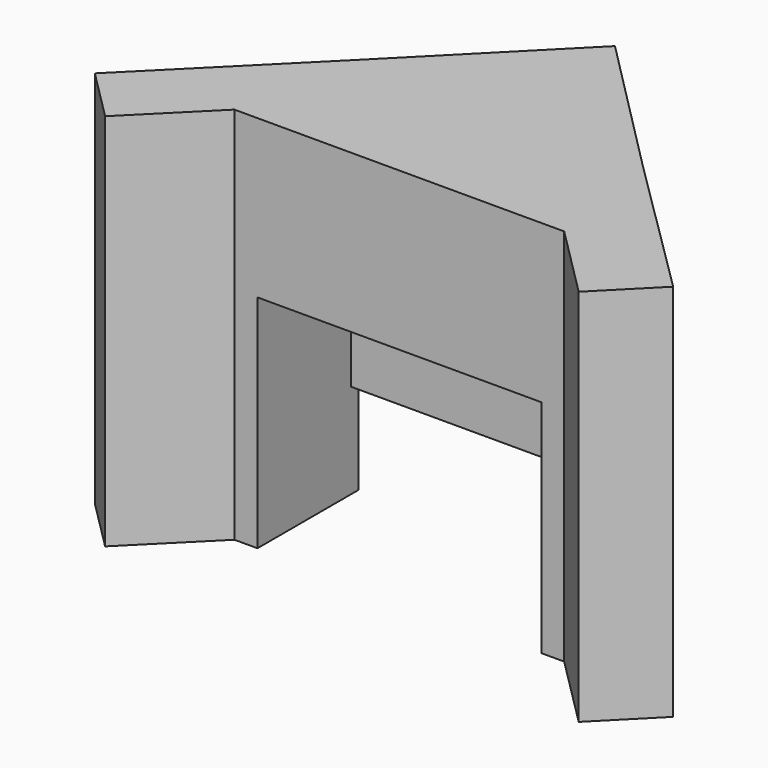
from build123d import *

# Parameters (mm, degrees)
F1_DEPTH = 15
F3_DEPTH = 60
F4_DEPTH = 35
F5_DEPTH = 15


# Not quite as in the source:
# - a feature of the source that left no trace in its solid (it failed there, or was rolled back) is left out


with BuildPart() as f1:
    # F0 (on Top) → F1 (new body)
    with BuildSketch(Plane.XY):
        Polygon((-45.7041380099, -77.9803808107), (-37.5291732437, -86.155345577), (-26.1500704675, -74.7762428008), (-22.5, -74.7762428008), (-22.5, -56.2421455979), (-22.5, -54.7762428008), align=None)
    extrude(amount=F1_DEPTH)


with BuildPart() as f1b:
    # F0 (on Top) → F1, piece 2 (new body)
    with BuildSketch(Plane.XY):
        Polygon((26.0955594839, -74.7762428008), (37.5969056221, -86.277588939), (45.8779636159, -77.9177674474), (22.4999970904, -54.7600604596), (22.5005300594, -56.2421455979), (22.5071950618, -74.7762428008), align=None)
    extrude(amount=F1_DEPTH)


with BuildPart() as f3:
    # F0 (on Top) → F3 (new body)
    with BuildSketch(Plane.XY):
        Polygon((-45.7041380099, -77.9803808107), (-37.5291732437, -86.155345577), (-26.1500704675, -74.7762428008), (-22.5, -74.7762428008), (-22.5, -56.2421455979), (-22.5, -54.7762428008), align=None)
        Polygon((-22.5, -56.2421455979), (-22.5, -74.7762428008), (0, -74.7762428008), (-0.0066650023, -56.2421455979), align=None)
        Polygon((0, -74.7762428008), (22.5071950618, -74.7762428008), (22.5005300594, -56.2421455979), (-0.0066650023, -56.2421455979), align=None)
        Polygon((26.0955594839, -74.7762428008), (37.5969056221, -86.277588939), (45.8779636159, -77.9177674474), (22.4999970904, -54.7600604596), (22.5005300594, -56.2421455979), (22.5071950618, -74.7762428008), align=None)
        Polygon((-0.0071950608, -54.7681542171), (-22.5, -54.7762428008), (-22.5, -56.2421455979), (-0.0066650023, -56.2421455979), align=None)
        Polygon((22.5005300594, -56.2421455979), (22.4999970904, -54.7600604596), (-0.0071950608, -54.7681542171), (-0.0066650023, -56.2421455979), align=None)
        Polygon((-0.0153547065, -32.0777396508), (-22.5, -54.7762428008), (-0.0071950608, -54.7681542171), align=None)
        Polygon((-0.0071950608, -54.7681542171), (22.4999970904, -54.7600604596), (-0.0153547065, -32.0777396508), align=None)
    extrude(amount=F3_DEPTH)

    # F0 (on Top) → F4 (cut)
    with BuildSketch(Plane.XY):
        Polygon((-22.5, -56.2421455979), (-22.5, -74.7762428008), (0, -74.7762428008), (-0.0066650023, -56.2421455979), align=None)
        Polygon((0, -74.7762428008), (22.5071950618, -74.7762428008), (22.5005300594, -56.2421455979), (-0.0066650023, -56.2421455979), align=None)
    extrude(amount=F4_DEPTH, mode=Mode.SUBTRACT)

    # F0 (on Top) → F5 (cut)
    with BuildSketch(Plane.XY):
        Polygon((-0.0071950608, -54.7681542171), (-22.5, -54.7762428008), (-22.5, -56.2421455979), (-0.0066650023, -56.2421455979), align=None)
        Polygon((22.5005300594, -56.2421455979), (22.4999970904, -54.7600604596), (-0.0071950608, -54.7681542171), (-0.0066650023, -56.2421455979), align=None)
        Polygon((-0.0071950608, -54.7681542171), (22.4999970904, -54.7600604596), (-0.0153547065, -32.0777396508), align=None)
        Polygon((-0.0153547065, -32.0777396508), (-22.5, -54.7762428008), (-0.0071950608, -54.7681542171), align=None)
    extrude(amount=F5_DEPTH, mode=Mode.SUBTRACT)


solid = Compound([f1.part, f1b.part, f3.part])
